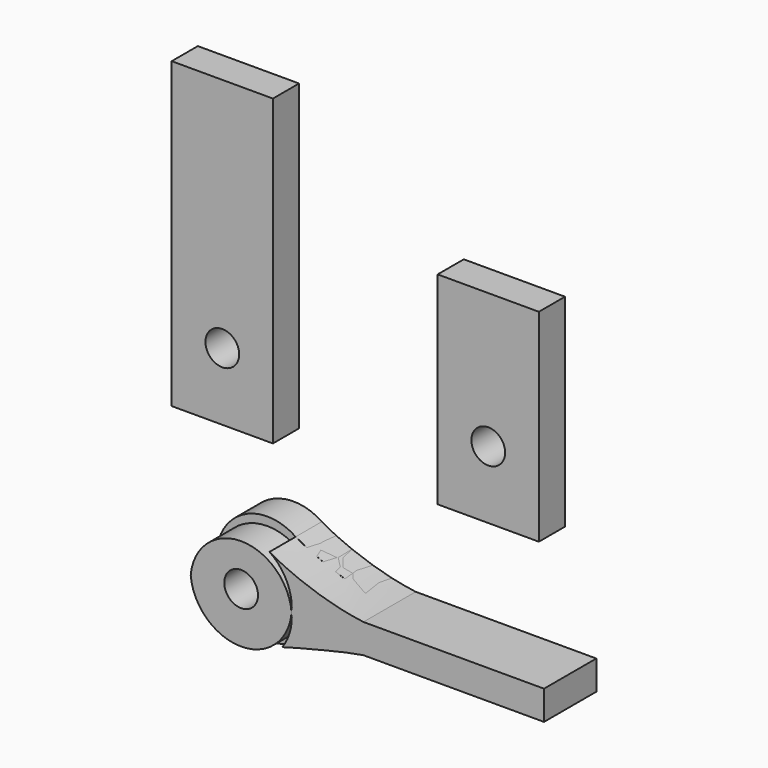
from build123d import *

# Parameters (mm, degrees)
F0_W     = 38.1
F0_H     = 114.3
F0_R     = 6.35
F1_DEPTH = 12.2936
F0_H_2   = 76.2
F2_DEPTH = 24.6126


with BuildPart() as f1:
    # F0 (on Front) → F1 (new body)
    with BuildSketch(Plane.XZ):
        with Locations((-16.9488759977, 31.75)):
            Rectangle(F0_W, F0_H)
        with Locations((-16.9488759977, 0)):
            Circle(F0_R, mode=Mode.SUBTRACT)
    extrude(amount=F1_DEPTH)


with BuildPart() as f1b:
    # F0 (on Front) → F1, piece 2 (new body)
    with BuildSketch(Plane.XZ):
        with Locations((83.1626755297, 12.7)):
            Rectangle(F0_W, F0_H_2)
        with Locations((83.1626755297, 0)):
            Circle(F0_R, mode=Mode.SUBTRACT)
    extrude(amount=F1_DEPTH)


with BuildPart() as f1c:
    # F0 (on Front) → F1, piece 3 (new body)
    with BuildSketch(Plane.XZ):
        with BuildLine():
            ThreePointArc((18.9837389297, -70.8980097773), (19.0334275238, -70.1049508984), (19.05, -69.3105097773))
            ThreePointArc((19.05, -69.3105097773), (18.9406359278, -67.2721745126), (18.6137994067, -65.2572429901))
            ThreePointArc((18.6137994067, -65.2572429901), (15.7729984646, -58.6280466047), (10.6713850071, -53.5300141568))
            ThreePointArc((10.6713850071, -53.5300141568), (-9.6273373734, -52.8722350778), (-18.9837389297, -70.8980097773))
            ThreePointArc((-18.9837389297, -70.8980097773), (0, -53.4355097773), (18.9837389297, -70.8980097773))
        make_face()
        with BuildLine():
            ThreePointArc((17.7329124706, -76.2708485126), (18.5538398056, -73.6299459059), (18.9837389297, -70.8980097773))
            ThreePointArc((18.9837389297, -70.8980097773), (0, -53.4355097773), (-18.9837389297, -70.8980097773))
            ThreePointArc((-18.9837389297, -70.8980097773), (-8.2239946562, -86.4938858104), (10.6713850071, -85.0910053979))
            ThreePointArc((10.6713850071, -85.0910053979), (14.871106908, -81.2165031978), (17.7329124706, -76.2708485126))
        make_face()
        with Locations((0, -69.3105097773)):
            Circle(F0_R, mode=Mode.SUBTRACT)
        with BuildLine():
            Line((18.6701288335, -76.2708485126), (17.7329124706, -76.2708485126))
            ThreePointArc((17.7329124706, -76.2708485126), (14.871106908, -81.2165031978), (10.6713850071, -85.0910053979))
            add(Edge.make_bspline(
                [(10.6713850071, -85.0910053979), (12.1969107154, -84.5431198491), (13.8321735998, -84.0204148681), (15.529884584, -83.5184234817)],
                knots=[0, 0, 0, 0, 0.1459300345, 0.1459300345, 0.1459300345, 0.1459300345], degree=3))
            ThreePointArc((15.529884584, -83.5184234817), (17.479761588, -80.0591769754), (18.6701288335, -76.2708485126))
        make_face()
        with BuildLine():
            ThreePointArc((10.6713850071, -85.0910053979), (-8.2239946562, -86.4938858104), (-18.9837389297, -70.8980097773))
            ThreePointArc((-18.9837389297, -70.8980097773), (-6.5422464015, -90.3768907196), (15.529884584, -83.5184234817))
            add(Edge.make_bspline(
                [(10.6713850071, -85.0910053979), (12.1969107154, -84.5431198491), (13.8321735998, -84.0204148681), (15.529884584, -83.5184234817)],
                knots=[0, 0, 0, 0, 0.1459300345, 0.1459300345, 0.1459300345, 0.1459300345], degree=3))
        make_face()
        with BuildLine():
            ThreePointArc((19.05, -72.4855097773), (19.0334275238, -71.6910686563), (18.9837389297, -70.8980097773))
            ThreePointArc((18.9837389297, -70.8980097773), (18.5538398056, -73.6299459059), (17.7329124706, -76.2708485126))
            Line((17.7329124706, -76.2708485126), (18.6701288335, -76.2708485126))
            ThreePointArc((18.6701288335, -76.2708485126), (18.9547943048, -74.3876856002), (19.05, -72.4855097773))
        make_face()
        with BuildLine():
            ThreePointArc((10.6713850071, -53.5300141568), (15.7729984646, -58.6280466047), (18.6137994067, -65.2572429901))
            Line((18.6137994067, -65.2572429901), (46.010632673, -65.2572429901))
            add(Edge.make_bspline(
                [(10.6713850071, -53.5300141568), (15.855355067, -56.5924877327), (28.7587196398, -61.8513925035), (39.4621942281, -64.3479001906), (46.010632673, -65.2572429901)],
                knots=[0, 0, 0, 0, 0.5085766586, 1, 1, 1, 1], degree=3))
        make_face()
        with BuildLine():
            ThreePointArc((18.6137994067, -65.2572429901), (18.9406359278, -67.2721745126), (19.05, -69.3105097773))
            ThreePointArc((19.05, -69.3105097773), (19.0334275238, -70.1049508984), (18.9837389297, -70.8980097773))
            ThreePointArc((18.9837389297, -70.8980097773), (19.0334275238, -71.6910686563), (19.05, -72.4855097773))
            ThreePointArc((19.05, -72.4855097773), (18.9547943048, -74.3876856002), (18.6701288335, -76.2708485126))
            Line((18.6701288335, -76.2708485126), (46.010632673, -76.2708485126))
            Line((46.010632673, -76.2708485126), (113.9992779968, -76.2708485126))
            Line((113.9992779968, -76.2708485126), (113.9992779968, -65.2572429901))
            Line((113.9992779968, -65.2572429901), (46.010632673, -65.2572429901))
            Line((46.010632673, -65.2572429901), (18.6137994067, -65.2572429901))
        make_face()
        with BuildLine():
            Line((46.010632673, -76.2708485126), (18.6701288335, -76.2708485126))
            ThreePointArc((18.6701288335, -76.2708485126), (17.479761588, -80.0591769754), (15.529884584, -83.5184234817))
            add(Edge.make_bspline(
                [(15.529884584, -83.5184234817), (19.680689102, -82.291083767), (30.5102969423, -79.6495257935), (39.5186451666, -77.343375938), (46.010632673, -76.2708485126)],
                knots=[0.1459300345, 0.1459300345, 0.1459300345, 0.1459300345, 0.5027204729, 1, 1, 1, 1], degree=3))
        make_face()
    extrude(amount=F1_DEPTH)


with BuildPart() as f2:
    # F0 (on Front) → F2 (new body)
    with BuildSketch(Plane.XZ):
        with BuildLine():
            ThreePointArc((18.6137994067, -65.2572429901), (18.9406359278, -67.2721745126), (19.05, -69.3105097773))
            ThreePointArc((19.05, -69.3105097773), (19.0334275238, -70.1049508984), (18.9837389297, -70.8980097773))
            ThreePointArc((18.9837389297, -70.8980097773), (19.0334275238, -71.6910686563), (19.05, -72.4855097773))
            ThreePointArc((19.05, -72.4855097773), (18.9547943048, -74.3876856002), (18.6701288335, -76.2708485126))
            Line((18.6701288335, -76.2708485126), (46.010632673, -76.2708485126))
            Line((46.010632673, -76.2708485126), (113.9992779968, -76.2708485126))
            Line((113.9992779968, -76.2708485126), (113.9992779968, -65.2572429901))
            Line((113.9992779968, -65.2572429901), (46.010632673, -65.2572429901))
            Line((46.010632673, -65.2572429901), (18.6137994067, -65.2572429901))
        make_face()
        with BuildLine():
            ThreePointArc((10.6713850071, -53.5300141568), (15.7729984646, -58.6280466047), (18.6137994067, -65.2572429901))
            Line((18.6137994067, -65.2572429901), (46.010632673, -65.2572429901))
            add(Edge.make_bspline(
                [(10.6713850071, -53.5300141568), (15.855355067, -56.5924877327), (28.7587196398, -61.8513925035), (39.4621942281, -64.3479001906), (46.010632673, -65.2572429901)],
                knots=[0, 0, 0, 0, 0.5085766586, 1, 1, 1, 1], degree=3))
        make_face()
        with BuildLine():
            Line((46.010632673, -76.2708485126), (18.6701288335, -76.2708485126))
            ThreePointArc((18.6701288335, -76.2708485126), (17.479761588, -80.0591769754), (15.529884584, -83.5184234817))
            add(Edge.make_bspline(
                [(15.529884584, -83.5184234817), (19.680689102, -82.291083767), (30.5102969423, -79.6495257935), (39.5186451666, -77.343375938), (46.010632673, -76.2708485126)],
                knots=[0.1459300345, 0.1459300345, 0.1459300345, 0.1459300345, 0.5027204729, 1, 1, 1, 1], degree=3))
        make_face()
    extrude(amount=F2_DEPTH)


with BuildPart() as f2b:
    # F0 (on Front) → F2, piece 2 (new body)
    with BuildSketch(Plane.XZ):
        with BuildLine():
            ThreePointArc((17.7329124706, -76.2708485126), (18.5538398056, -73.6299459059), (18.9837389297, -70.8980097773))
            ThreePointArc((18.9837389297, -70.8980097773), (0, -53.4355097773), (-18.9837389297, -70.8980097773))
            ThreePointArc((-18.9837389297, -70.8980097773), (-8.2239946562, -86.4938858104), (10.6713850071, -85.0910053979))
            ThreePointArc((10.6713850071, -85.0910053979), (14.871106908, -81.2165031978), (17.7329124706, -76.2708485126))
        make_face()
        with Locations((0, -69.3105097773)):
            Circle(F0_R, mode=Mode.SUBTRACT)
    extrude(amount=F2_DEPTH)


solid = Compound([f1.part, f1b.part, f1c.part, f2.part, f2b.part])
